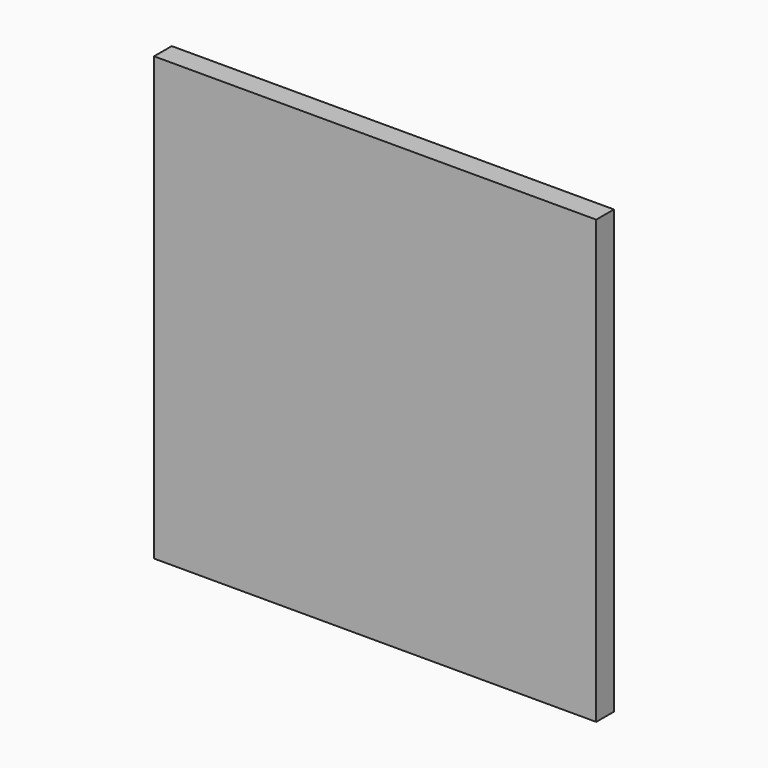
from build123d import *

# Parameters (mm, degrees)
F0_W     = 63.5
F0_H     = 63.5
F1_DEPTH = 3.175


# Not quite as in the source:
# - a length typed as a fraction of an inch, garbled in the dataset ("3 / 203.2 mm" for 3/8 in), is restored


with BuildPart() as f1:
    # F0 (on Front) → F1 (new body)
    with BuildSketch(Plane.XZ):
        Rectangle(F0_W, F0_H)
    extrude(amount=F1_DEPTH)


solid = f1.part
